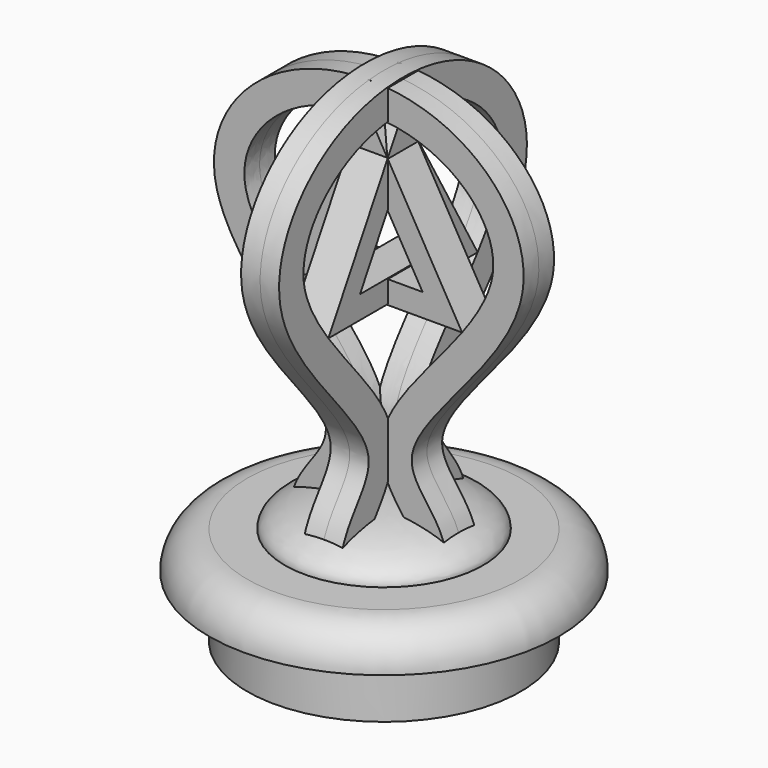
from build123d import *

# Parameters (mm, degrees)
F3_DEPTH      = 2.5
F3_DEPTH_BACK = 2.5
F5_DEPTH      = 2.5
F5_DEPTH_BACK = 2.5
F6_W          = 5
F6_H          = 13
F7_DEPTH      = 10


# Not quite as in the source:
# - ends of sketch curves that miss each other by under 0.0002 mm in the source are joined
# - the dataset's text gives a spline's control points without its knots; the knots are read off the source's solid


with BuildPart() as f1:
    # F0 (on Front) → F1 (revolve)
    with BuildSketch(Plane.XZ):
        with BuildLine():
            Line((-18, 0), (0, 0))
            Line((0, 0), (0, 13))
            Line((0, 13), (0, 17.2006769083))
            add(Edge.make_bspline(
                [(0, 17.2006769083), (-13.0361616611, 17.2006769083), (-13.0361616611, 13)],
                knots=[4.7123889804, 4.7123889804, 4.7123889804, 6.2831853072, 6.2831853072, 6.2831853072], degree=2, weights=[1, 0.7071067812, 1]))
            Line((-13.0361616611, 13), (-18, 13))
            ThreePointArc((-18, 13), (-21.5355339059, 11.5355339059), (-23, 8))
            Line((-23, 8), (-18, 8))
            Line((-18, 8), (-18, 0))
        make_face()
    revolve(axis=Axis((0, 0, 6.5), (0, 0, 1)))

    # F2 (on Front) → F3 (join, two sides)
    with BuildSketch(Plane.XZ) as f3_sk:
        with BuildLine():
            add(Edge.make_bspline(
                [(-10.4089388328, 13.049096218), (-10.1139522415, 18.3864439428), (1.9570521569, 23.7888203331), (-30.8524401677, 47.5172177819), (-12.8202655471, 66), (0, 66)],
                knots=[0.0044055008, 0.0044055008, 0.0044055008, 0.0044055008, 0.250996542, 0.6272609792, 1, 1, 1, 1], degree=3))
            Line((-10.4089388328, 13.049096218), (-6.3983946003, 13.049096218))
            add(Edge.make_bspline(
                [(-6.3983946003, 13.049096218), (-6.3747748228, 13.2899927496), (-6.2748477492, 13.8474801838), (-5.979471531, 14.6723165704), (-5.4293029105, 15.6649356099), (-4.6582444134, 16.7730916079), (-3.7197607843, 18.0488708512), (-2.8712739404, 19.3556366184), (-2.2540858272, 20.6553730602), (-1.8745159631, 21.780012764), (-1.6840483914, 22.8387492488), (-1.6393589038, 23.7336535308), (-1.6601104568, 24.3053967184), (-1.7069052403, 24.7633460073), (-1.7712616023, 25.2085995493), (-1.8816295367, 25.7461035666), (-2.0528756582, 26.3609018119), (-2.3237504947, 27.1454363858), (-2.7283269426, 28.0698501884), (-3.2920966049, 29.1194883122), (-3.9191628431, 30.1327771372), (-4.8259840471, 31.4566452027), (-6.0713945434, 33.0888164216), (-7.6822252046, 35.055464985), (-9.3427786709, 37.0416940528), (-10.8991617523, 38.9432394165), (-11.853999899, 40.177808921), (-12.2730990884, 40.7423673653)],
                knots=[0.0105707221, 0.0105707221, 0.0105707221, 0.0105707221, 0.03125, 0.0625, 0.09375, 0.125, 0.15625, 0.1875, 0.203125, 0.21875, 0.234375, 0.2421875, 0.25, 0.25390625, 0.2578125, 0.265625, 0.2734375, 0.28125, 0.296875, 0.3125, 0.328125, 0.34375, 0.375, 0.40625, 0.4375, 0.46875, 0.4952985245, 0.4952985245, 0.4952985245, 0.4952985245], degree=3))
            add(Edge.make_bspline(
                [(-12.2730990884, 40.7423673653), (-12.3473173207, 40.8423449622), (-12.9101801431, 41.606255514), (-13.8907684674, 43.0239877246), (-15.0117097717, 44.9403794429), (-15.687161828, 46.4443285256), (-16.0548171196, 47.5643144646), (-16.2125446126, 48.2245948008), (-16.2969038177, 48.7298206348), (-16.3569906911, 49.2367486596), (-16.3864842126, 49.8685003764), (-16.3510692981, 50.6275955068), (-16.2100413683, 51.641876589), (-15.8573663697, 52.9146746714), (-15.1464670534, 54.4353735919), (-14.1456314239, 55.9190775738), (-12.4317310692, 57.7976257384), (-9.6057638872, 59.8573850216), (-5.2610015273, 61.5606522184), (-1.8288712343, 62), (0, 62)],
                knots=[0.4952985245, 0.4952985245, 0.4952985245, 0.4952985245, 0.5, 0.53125, 0.5625, 0.59375, 0.609375, 0.625, 0.6328125, 0.640625, 0.65625, 0.671875, 0.6875, 0.71875, 0.75, 0.78125, 0.8125, 0.875, 0.9375, 1, 1, 1, 1], degree=3))
            add(Edge.make_bspline(
                [(12.2730990884, 40.7423673653), (12.3473173207, 40.8423449622), (12.9101801431, 41.606255514), (13.8907684674, 43.0239877246), (15.0117097717, 44.9403794429), (15.687161828, 46.4443285256), (16.0548171196, 47.5643144646), (16.2125446126, 48.2245948008), (16.2969038177, 48.7298206348), (16.3569906911, 49.2367486596), (16.3864842126, 49.8685003764), (16.3510692981, 50.6275955068), (16.2100413683, 51.641876589), (15.8573663697, 52.9146746714), (15.1464670534, 54.4353735919), (14.1456314239, 55.9190775738), (12.4317310692, 57.7976257384), (9.6057638872, 59.8573850216), (5.2610015273, 61.5606522184), (1.8288712343, 62), (0, 62)],
                knots=[0.4952985245, 0.4952985245, 0.4952985245, 0.4952985245, 0.5, 0.53125, 0.5625, 0.59375, 0.609375, 0.625, 0.6328125, 0.640625, 0.65625, 0.671875, 0.6875, 0.71875, 0.75, 0.78125, 0.8125, 0.875, 0.9375, 1, 1, 1, 1], degree=3))
            add(Edge.make_bspline(
                [(6.3996669298, 13.0359732788), (6.3762174502, 13.2819174756), (6.2761829449, 13.8437516577), (5.979471531, 14.6723165704), (5.4293029105, 15.6649356099), (4.6582444134, 16.7730916079), (3.7197607843, 18.0488708512), (2.8712739404, 19.3556366184), (2.2540858272, 20.6553730602), (1.8745159631, 21.780012764), (1.6840483914, 22.8387492488), (1.6393589038, 23.7336535308), (1.6601104568, 24.3053967184), (1.7069052403, 24.7633460073), (1.7712616023, 25.2085995493), (1.8816295367, 25.7461035666), (2.0528756582, 26.3609018119), (2.3237504947, 27.1454363858), (2.7283269426, 28.0698501884), (3.2920966049, 29.1194883122), (3.9191628431, 30.1327771372), (4.8259840471, 31.4566452027), (6.0713945434, 33.0888164216), (7.6822252046, 35.055464985), (9.3427786709, 37.0416940528), (10.8991617523, 38.9432394165), (11.853999899, 40.177808921), (12.2730990884, 40.7423673653)],
                knots=[0.010194725, 0.010194725, 0.010194725, 0.010194725, 0.03125, 0.0625, 0.09375, 0.125, 0.15625, 0.1875, 0.203125, 0.21875, 0.234375, 0.2421875, 0.25, 0.25390625, 0.2578125, 0.265625, 0.2734375, 0.28125, 0.296875, 0.3125, 0.328125, 0.34375, 0.375, 0.40625, 0.4375, 0.46875, 0.4952985245, 0.4952985245, 0.4952985245, 0.4952985245], degree=3))
            Line((6.3996669298, 13.0359732788), (10.4096564485, 13.0359413301))
            add(Edge.make_bspline(
                [(10.4096564485, 13.0359413301), (10.1218042481, 18.3829323182), (-1.9637251545, 23.7839943048), (30.8524401677, 47.5172177819), (12.8202655471, 66), (0, 66)],
                knots=[0.0042030107, 0.0042030107, 0.0042030107, 0.0042030107, 0.250996542, 0.6272609792, 1, 1, 1, 1], degree=3))
        make_face()
    extrude(amount=F3_DEPTH)
    extrude(f3_sk.sketch, amount=-F3_DEPTH_BACK)

    # F6 (on face) → F7 (cut)
    with BuildSketch(Plane(origin=(0, 0, 0), x_dir=(1, 0, 0), z_dir=(0, 0, -1))):
        Rectangle(F6_W, F6_H)
    extrude(amount=-F7_DEPTH, mode=Mode.SUBTRACT)


with BuildPart() as f3:
    # F2 (on Front) → F3, piece 2 (new body, two sides)
    with BuildSketch(Plane.XZ) as f3_2_sk:
        Polygon((0, 62), (-12.2731005508, 40.7423662797), (12.2731005508, 40.7423662797), align=None)
        Polygon((7.0769481281, 43.7423662797), (-7.0769481281, 43.7423662797), (0, 56), align=None, mode=Mode.SUBTRACT)
    extrude(amount=F3_DEPTH)
    extrude(f3_2_sk.sketch, amount=-F3_DEPTH_BACK)


with BuildPart() as f5:
    # F4 (on Right) → F5 (new body, two sides)
    with BuildSketch(Plane.YZ) as f5_sk:
        with BuildLine():
            add(Edge.make_bspline(
                [(-10.4082621174, 13.1723851922), (-10.106729356, 18.500868019), (1.9509086382, 23.9044527549), (-30.8524401677, 47.6284071038), (-12.8202655471, 66.1111893219), (0, 66.1111893219)],
                knots=[0.0045919241, 0.0045919241, 0.0045919241, 0.0045919241, 0.250996542, 0.6272609792, 1, 1, 1, 1], degree=3))
            Line((-10.4082621174, 13.1723851922), (-6.3971926816, 13.1723851922))
            add(Edge.make_bspline(
                [(-6.3971926816, 13.1723851922), (-6.3734364264, 13.4086259933), (-6.27361629, 13.9621083486), (-5.979471531, 14.7835058923), (-5.4293029105, 15.7761249319), (-4.6582444134, 16.8842809298), (-3.7197607843, 18.1600601731), (-2.8712739404, 19.4668259403), (-2.2540858272, 20.7665623821), (-1.8745159631, 21.8912020859), (-1.6840483914, 22.9499385707), (-1.6393589038, 23.8448428527), (-1.6601104568, 24.4165860404), (-1.7069052403, 24.8745353293), (-1.7712616023, 25.3197888712), (-1.8816295367, 25.8572928885), (-2.0528756582, 26.4720911338), (-2.3237504947, 27.2566257077), (-2.7283269426, 28.1810395104), (-3.2920966049, 29.2306776341), (-3.9191628431, 30.2439664591), (-4.8259840471, 31.5678345246), (-6.0713945434, 33.2000057436), (-7.6822252046, 35.1666543069), (-9.3427786709, 37.1528833747), (-10.8991617523, 39.0544287385), (-11.853999899, 40.288998243), (-12.2730990884, 40.8535566872)],
                knots=[0.0109175066, 0.0109175066, 0.0109175066, 0.0109175066, 0.03125, 0.0625, 0.09375, 0.125, 0.15625, 0.1875, 0.203125, 0.21875, 0.234375, 0.2421875, 0.25, 0.25390625, 0.2578125, 0.265625, 0.2734375, 0.28125, 0.296875, 0.3125, 0.328125, 0.34375, 0.375, 0.40625, 0.4375, 0.46875, 0.4952985245, 0.4952985245, 0.4952985245, 0.4952985245], degree=3))
            add(Edge.make_bspline(
                [(-12.2730990884, 40.8535566872), (-12.3473173207, 40.9535342841), (-12.9101801431, 41.717444836), (-13.8907684674, 43.1351770465), (-15.0117097717, 45.0515687649), (-15.687161828, 46.5555178476), (-16.0548171196, 47.6755037865), (-16.2125446126, 48.3357841227), (-16.2969038177, 48.8410099567), (-16.3569906911, 49.3479379816), (-16.3864842126, 49.9796896983), (-16.3510692981, 50.7387848288), (-16.2100413683, 51.7530659109), (-15.8573663697, 53.0258639934), (-15.1464670534, 54.5465629138), (-14.1456314239, 56.0302668958), (-12.4317310692, 57.9088150603), (-9.6057638872, 59.9685743436), (-5.2610015273, 61.6718415404), (-1.8288712343, 62.1111893219), (0, 62.1111893219)],
                knots=[0.4952985245, 0.4952985245, 0.4952985245, 0.4952985245, 0.5, 0.53125, 0.5625, 0.59375, 0.609375, 0.625, 0.6328125, 0.640625, 0.65625, 0.671875, 0.6875, 0.71875, 0.75, 0.78125, 0.8125, 0.875, 0.9375, 1, 1, 1, 1], degree=3))
            add(Edge.make_bspline(
                [(12.2730990884, 40.8535566872), (12.3473173207, 40.9535342841), (12.9101801431, 41.717444836), (13.8907684674, 43.1351770465), (15.0117097717, 45.0515687649), (15.687161828, 46.5555178476), (16.0548171196, 47.6755037865), (16.2125446126, 48.3357841227), (16.2969038177, 48.8410099567), (16.3569906911, 49.3479379816), (16.3864842126, 49.9796896983), (16.3510692981, 50.7387848288), (16.2100413683, 51.7530659109), (15.8573663697, 53.0258639934), (15.1464670534, 54.5465629138), (14.1456314239, 56.0302668958), (12.4317310692, 57.9088150603), (9.6057638872, 59.9685743436), (5.2610015273, 61.6718415404), (1.8288712343, 62.1111893219), (0, 62.1111893219)],
                knots=[0.4952985245, 0.4952985245, 0.4952985245, 0.4952985245, 0.5, 0.53125, 0.5625, 0.59375, 0.609375, 0.625, 0.6328125, 0.640625, 0.65625, 0.671875, 0.6875, 0.71875, 0.75, 0.78125, 0.8125, 0.875, 0.9375, 1, 1, 1, 1], degree=3))
            add(Edge.make_bspline(
                [(6.4007248036, 13.1359311522), (6.3774386891, 13.3862281804), (6.2773196996, 13.9517665985), (5.979471531, 14.7835058923), (5.4293029105, 15.7761249319), (4.6582444134, 16.8842809298), (3.7197607843, 18.1600601731), (2.8712739404, 19.4668259403), (2.2540858272, 20.7665623821), (1.8745159631, 21.8912020859), (1.6840483914, 22.9499385707), (1.6393589038, 23.8448428527), (1.6601104568, 24.4165860404), (1.7069052403, 24.8745353293), (1.7712616023, 25.3197888712), (1.8816295367, 25.8572928885), (2.0528756582, 26.4720911338), (2.3237504947, 27.2566257077), (2.7283269426, 28.1810395104), (3.2920966049, 29.2306776341), (3.9191628431, 30.2439664591), (4.8259840471, 31.5678345246), (6.0713945434, 33.2000057436), (7.6822252046, 35.1666543069), (9.3427786709, 37.1528833747), (10.8991617523, 39.0544287385), (11.853999899, 40.288998243), (12.2730990884, 40.8535566872)],
                knots=[0.0098746097, 0.0098746097, 0.0098746097, 0.0098746097, 0.03125, 0.0625, 0.09375, 0.125, 0.15625, 0.1875, 0.203125, 0.21875, 0.234375, 0.2421875, 0.25, 0.25390625, 0.2578125, 0.265625, 0.2734375, 0.28125, 0.296875, 0.3125, 0.328125, 0.34375, 0.375, 0.40625, 0.4375, 0.46875, 0.4952985245, 0.4952985245, 0.4952985245, 0.4952985245], degree=3))
            Line((6.4007248036, 13.1359311522), (10.4102541208, 13.1359010583))
            add(Edge.make_bspline(
                [(10.4102541208, 13.1359010583), (10.1285064022, 18.4911282717), (-1.9694163276, 23.891067671), (30.8524401677, 47.6284071038), (12.8202655471, 66.1111893219), (0, 66.1111893219)],
                knots=[0.0040303137, 0.0040303137, 0.0040303137, 0.0040303137, 0.250996542, 0.6272609792, 1, 1, 1, 1], degree=3))
        make_face()
    extrude(amount=F5_DEPTH)
    extrude(f5_sk.sketch, amount=-F5_DEPTH_BACK)


with BuildPart() as f5b:
    # F4 (on Right) → F5, piece 2 (new body, two sides)
    with BuildSketch(Plane.YZ) as f5_2_sk:
        Polygon((0, 62.1111893219), (-12.2731005508, 40.8535556016), (12.2731005508, 40.8535556016), align=None)
        Polygon((7.0769481281, 43.8535556016), (-7.0769481281, 43.8535556016), (0, 56.1111893219), align=None, mode=Mode.SUBTRACT)
    extrude(amount=F5_DEPTH)
    extrude(f5_2_sk.sketch, amount=-F5_DEPTH_BACK)


solid = Compound([f1.part, f3.part, f5.part, f5b.part])
